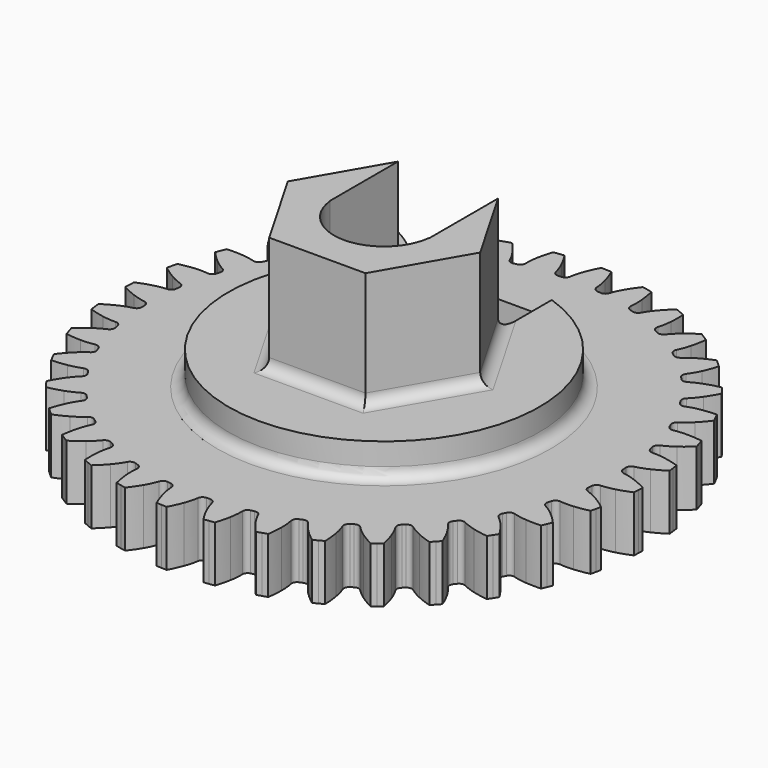
from build123d import *

# Parameters (mm, degrees)
F1_R            = 20.9375
F1_R_2          = 4.5
F2_DEPTH        = 5
F4_DEPTH        = 5
F4_COPIES_COUNT = 36
F5_R            = 4.5
F6_DEPTH        = 13.5
F7_R            = 14
F7_R_2          = 4.5
F8_DEPTH        = 3
F9_W            = 9
F9_H            = 16
F10_DEPTH       = 18.501
F11_R           = 1


# Not quite as in the source:
# - a pattern or mirror of a feature is missing from the dataset's text; its kind, count and spacing are read off the source's solid


with BuildPart() as f2:
    # F1 (on Top) → F2 (new body)
    with BuildSketch(Plane.XY):
        Circle(F1_R)
        Circle(F1_R_2, mode=Mode.SUBTRACT)
    extrude(amount=F2_DEPTH)

    # F3 (on Top) → F4 (join)
    with BuildSketch(Plane.XY):
        with BuildLine():
            ThreePointArc((1.0362892257, 23.7273809056), (0.802638016, 23.736433435), (0.5689090061, 23.7431851811))
            ThreePointArc((0.5689090061, 23.7431851811), (0.2618784806, 23.1319238772), (0, 22.5))
            ThreePointArc((0, 22.5), (0.9817476875, 22.4785713843), (1.9616253755, 22.4143263536))
            ThreePointArc((1.9616253755, 22.4143263536), (1.7558372948, 23.0666754864), (1.503267663, 23.7023772296))
            ThreePointArc((1.503267663, 23.7023772296), (1.2698399875, 23.7160284703), (1.0362892257, 23.7273809056))
        make_face()
        with BuildLine():
            ThreePointArc((1.9616253755, 22.4143263536), (0.9817476875, 22.4785713843), (0, 22.5))
            ThreePointArc((0, 22.5), (-0.185889302, 21.9168535458), (-0.3127105957, 21.3180789813))
            ThreePointArc((-0.3127105957, 21.3180789813), (-0.4650258761, 21.0410652431), (-0.7585808375, 20.9237535199))
            ThreePointArc((-0.7585808375, 20.9237535199), (0.9135707648, 20.9175594826), (2.5798953028, 20.7779461564))
            ThreePointArc((2.5798953028, 20.7779461564), (2.2976857448, 20.9204042946), (2.1701014237, 21.2096425991))
            ThreePointArc((2.1701014237, 21.2096425991), (2.0959662021, 21.8171939044), (1.9616253755, 22.4143263536))
        make_face()
    f4 = extrude(amount=F4_DEPTH)

    # F4_copies: F4 ×36 about axis
    f4_copies_axis = Axis((0, 0, 0), (0, 0, 1))
    for i in range(1, F4_COPIES_COUNT):
        add(f4.rotate(f4_copies_axis, i * 360 / F4_COPIES_COUNT))

    # F5 (on face) → F6 (join)
    with BuildSketch(Plane.XY.offset(5)):
        Polygon((8.6602540378, 0), (4.3301270189, 7.5), (-4.3301270189, 7.5), (-8.6602540378, 0), (-4.3301270189, -7.5), (4.3301270189, -7.5), align=None)
        Circle(F5_R, mode=Mode.SUBTRACT)
    extrude(amount=F6_DEPTH)

    # F7 (on face) → F8 (join)
    with BuildSketch(Plane.XY.offset(5)):
        Circle(F7_R)
        Circle(F7_R_2, mode=Mode.SUBTRACT)
    extrude(amount=F8_DEPTH)

    # F9 (on face) → F10 (cut, through all)
    with BuildSketch(Plane.XY.offset(18.5)):
        with Locations((0, 7.5)):
            Rectangle(F9_W, F9_H)
    extrude(amount=-F10_DEPTH, mode=Mode.SUBTRACT)

    # F11
    f11_edges = [f2.edges().sort_by_distance(p)[0] for p in [
        (-6.495191, -3.75, 8),
        (6.495191, -3.75, 8),
        (-6.580127, 3.602886, 8),
        (6.580127, 3.602886, 8),
        (0, -14, 5),
        (0, -7.5, 8),
    ]]
    fillet(f11_edges, radius=F11_R)


solid = f2.part
